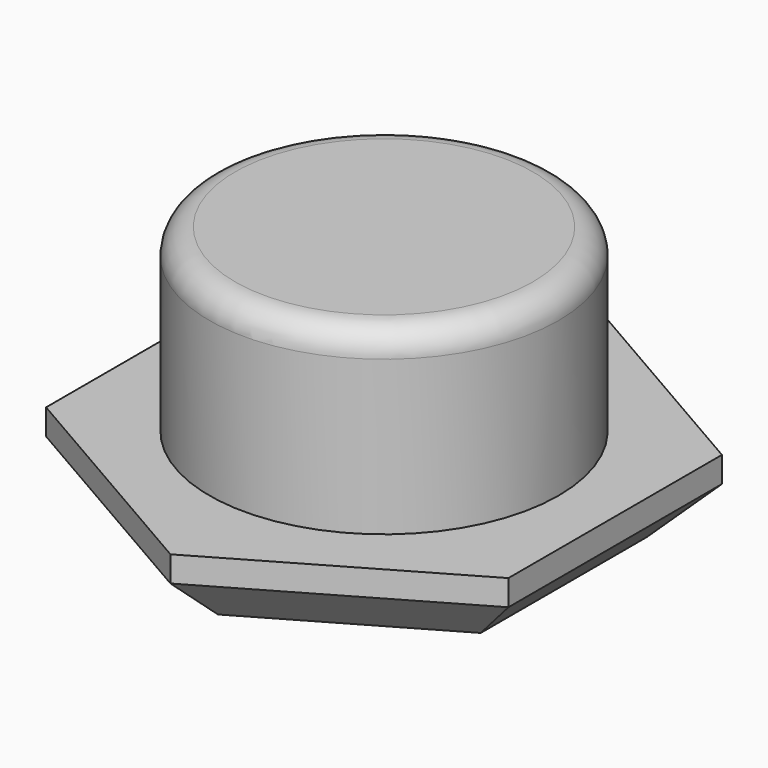
from build123d import *

# Parameters (mm, degrees)
F0_R     = 3.4
F1_DEPTH = 1.5
F0_R_2   = 1.5
F2_DEPTH = 5
F3_DEPTH = 2
F4_SIZE  = 1
F5_R     = 0.99999
F6_R     = 0.5


# Not quite as in the source:
# - a fillet or chamfer is up to 0.001 mm smaller than in the source, because OpenCascade refuses the exact size


with BuildPart() as f1:
    # F0 (on Top) → F1 (new body)
    with BuildSketch(Plane.XY):
        Polygon((4.5, -2.5980762114), (4.5, 2.5980762114), (0, 5.1961524227), (-4.5, 2.5980762114), (-4.5, -2.5980762114), (0, -5.1961524227), align=None)
        Circle(F0_R, mode=Mode.SUBTRACT)
    extrude(amount=F1_DEPTH)

    # F0 (on Top) → F2 (join)
    with BuildSketch(Plane.XY):
        Circle(F0_R)
        Circle(F0_R_2, mode=Mode.SUBTRACT)
        Circle(F0_R_2)
    extrude(amount=F2_DEPTH)

    # F0 (on Top) → F3 (cut)
    with BuildSketch(Plane.XY):
        Circle(F0_R_2)
    extrude(amount=F3_DEPTH, mode=Mode.SUBTRACT)

    # F4
    f4_edges = [f1.edges().sort_by_distance(p)[0] for p in [
        (4.5, 0, 0),
        (2.25, -3.897114, 0),
        (2.25, 3.897114, 0),
        (-2.25, -3.897114, 0),
        (-2.25, 3.897114, 0),
        (-4.5, 0, 0),
        (-1.5, 0, 0),
    ]]
    chamfer(f4_edges, length=F4_SIZE)

    # F5 (radius 1 in the source; OpenCascade refuses exactly that, so slightly less here)
    f5_edges = [f1.edges().sort_by_distance(p)[0] for p in [
        (-1.5, 0, 2),
    ]]
    fillet(f5_edges, radius=F5_R)

    # F6
    f6_edges = [f1.edges().sort_by_distance(p)[0] for p in [
        (-3.4, 0, 5),
    ]]
    fillet(f6_edges, radius=F6_R)


solid = f1.part
